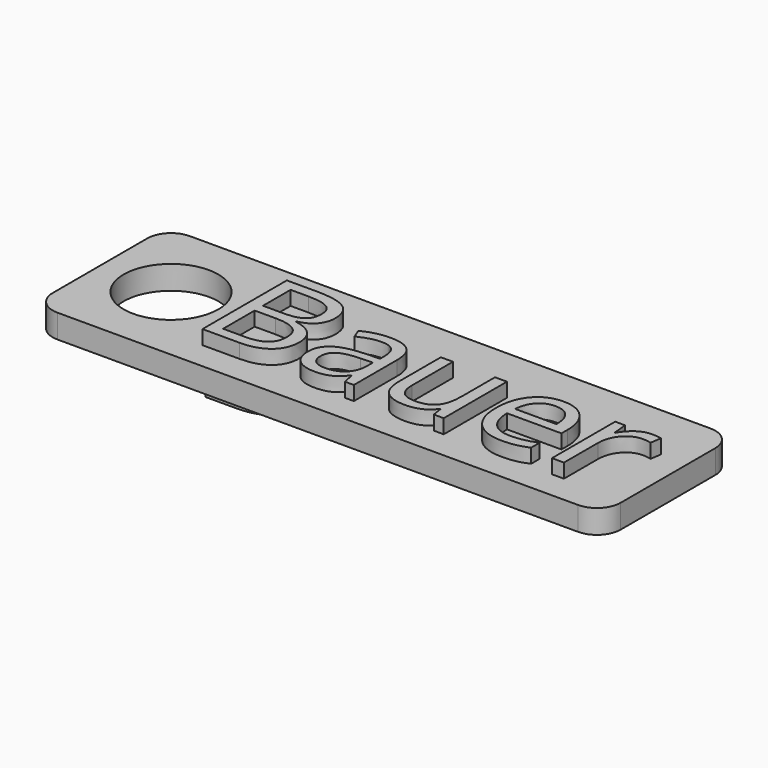
from build123d import *

# Parameters (mm, degrees)
F0_W         = 120
F0_H         = 35
F0_R         = 10
F1_DEPTH     = 5
F2_R         = 5
F3_TEXT_SIZE = 31.1975690743
F4_DEPTH     = 3
F5_TEXT_SIZE = 31.5927796894
F6_DEPTH     = 3


# Not quite as in the source:
# - Text() gives the source's letters only with a copy of the font that has no kerning and outlines rounded to 1/6400 em; it was checked with that copy


with BuildPart() as f1:
    # F0 (on Top) → F1 (new body)
    with BuildSketch(Plane.XY):
        Rectangle(F0_W, F0_H)
        with Locations((-45, 0)):
            Circle(F0_R, mode=Mode.SUBTRACT)
    extrude(amount=F1_DEPTH)

    # F2
    f2_edges = [f1.edges().sort_by_distance(p)[0] for p in [
        (-60, -17.5, 2.5),
        (60, -17.5, 2.5),
        (60, 17.5, 2.5),
        (-60, 17.5, 2.5),
    ]]
    fillet(f2_edges, radius=F2_R)

    # F3 (on face) → F4 (join)
    with BuildSketch(Plane.XY.offset(5)):
        with Locations((-32.1078058332, -11.6275176406)):
            Text('Bauer', F3_TEXT_SIZE, font='Open Sans', text_align=(TextAlign.LEFT, TextAlign.BOTTOM))
    extrude(amount=F4_DEPTH)

    # F5 (on face) → F6 (join)
    with BuildSketch(Plane(origin=(0, 0, 0), x_dir=(1, 0, 0), z_dir=(0, 0, -1))):
        with Locations((-29.8011898994, -8.7819928303)):
            Text('Ryan', F5_TEXT_SIZE, font='Open Sans', text_align=(TextAlign.LEFT, TextAlign.BOTTOM))
    extrude(amount=F6_DEPTH)


solid = f1.part
